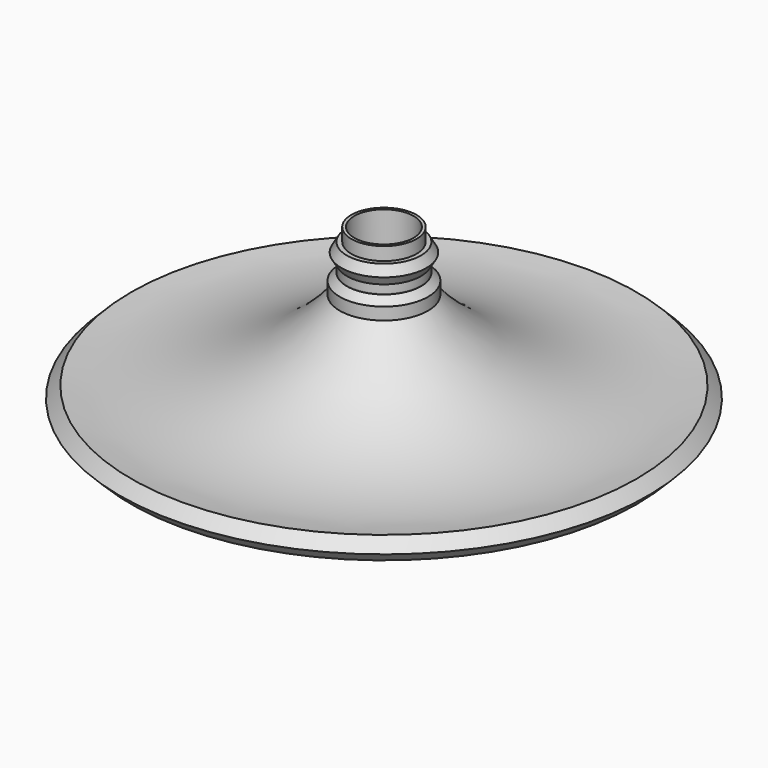
from build123d import *

# Parameters (mm, degrees)
F2_R        = 5.08
F3_S5_R     = 5.9685739689
F3_T6_DEPTH = 12
F4_R        = 4.7752
F5_DEPTH    = 14.605
F6_R        = 1.6002
F7_DEPTH    = 11.43
F8_R        = 1.5875
F9_DEPTH    = 11.43


# Not quite as in the source:
# - a fillet or chamfer that OpenCascade refuses, or shapes differently, is made with other operations: its cross-section is extruded or revolved along the edge and cut away or added


with BuildPart() as f1:
    # F0 (on Right) → F1 (revolve)
    with BuildSketch(Plane.YZ):
        with BuildLine():
            Line((0, 40.8495813608), (0, 0))
            Line((0, 0), (5.0717149861, 0))
            ThreePointArc((5.0717149861, 0), (20.9654737991, 11.9868064796), (40.676549077, 14.7740291432))
            Line((40.676549077, 14.7740291432), (42.4818582833, 16.5677014738))
            Line((42.4818582833, 16.5677014738), (40.676549077, 18.3847230526))
            ThreePointArc((40.676549077, 18.3847230526), (22.1270293001, 20.2430061627), (7.0992088877, 31.2748923898))
            Line((7.0992088877, 31.2748923898), (7.0992088877, 34.5178544521))
            Line((7.0992088877, 34.5178544521), (5.9685739689, 34.5178544521))
            Line((5.9685739689, 34.5178544521), (5.9685739689, 35.8129814267))
            Line((5.9685739689, 35.8129814267), (6.8319910206, 37.2520089149))
            Line((6.8319910206, 37.2520089149), (5.9685739689, 38.7390069664))
            Line((5.9685739689, 38.7390069664), (5.2490597591, 38.7390069664))
            Line((5.2490597591, 38.7390069664), (5.2490597591, 40.8495813608))
            Line((5.2490597591, 40.8495813608), (0, 40.8495813608))
        make_face()
    revolve(axis=Axis((0, 0, 20.4247906804), (0, 0, -1)))

    # F2
    f2_edges = [f1.edges().sort_by_distance(p)[0] for p in [
        (0, -5.071715, 0),
    ]]
    fillet(f2_edges, radius=F2_R)

    # F3: chamfer of 1.27 on 1 edges, made by hand


with BuildPart() as f3_tool2:
    # F3_s3 → F3_t4 (revolve)
    with BuildSketch(Plane.YZ):
        Polygon((7.0992088877, 33.2478544521), (5.8292088877, 34.5178544521), (7.0992088877, 34.5178544521), align=None)
    revolve(axis=Axis((0, 0, 34.5178544521), (0, 0, -1)))

    # F3_s5 → F3_t6 (cut, symmetric)
    with BuildSketch(Plane.XY.offset(33.9)):
        Circle(F3_S5_R)
    extrude(amount=F3_T6_DEPTH, both=True, mode=Mode.SUBTRACT)


with BuildPart() as f1_1:
    add(f1.part)

    # F3_t1: cut F3_tool2
    add(f3_tool2.part, mode=Mode.SUBTRACT)

    # F4 (on face) → F5 (cut)
    with BuildSketch(Plane.XY.offset(40.8495813608)):
        Circle(F4_R)
    extrude(amount=-F5_DEPTH, mode=Mode.SUBTRACT)

    # F6 (on face) → F7 (join)
    with BuildSketch(Plane(origin=(0, 0, 0), x_dir=(1, 0, 0), z_dir=(0, 0, -1))):
        Circle(F6_R)
    extrude(amount=-F7_DEPTH)

    # F8 (on Top) → F9 (cut)
    with BuildSketch(Plane.XY):
        Circle(F8_R)
    extrude(amount=F9_DEPTH, mode=Mode.SUBTRACT)


solid = f1_1.part
